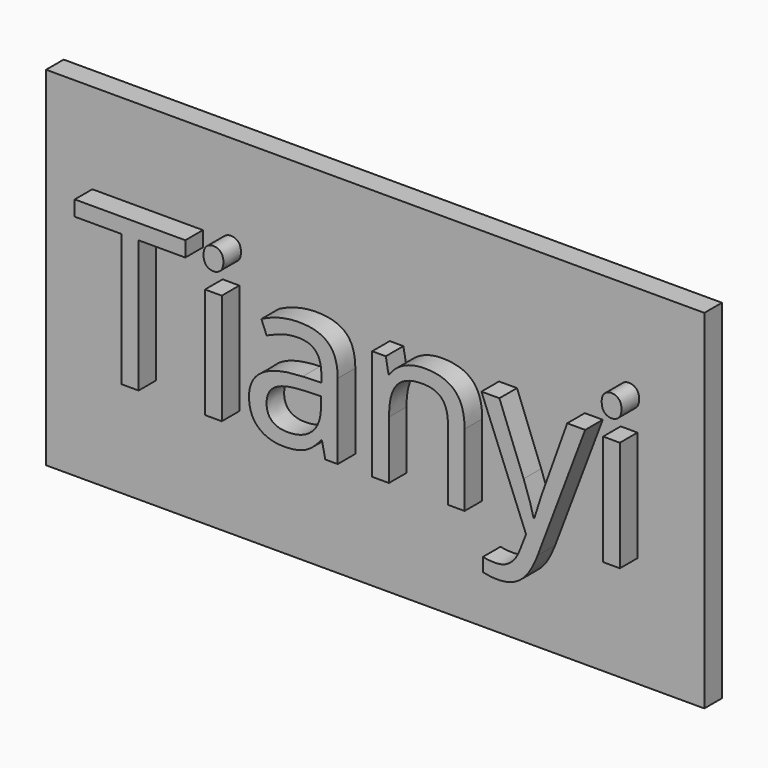
from build123d import *

# Parameters (mm, degrees)
F0_W         = 76.0509371758
F0_H         = 40.2351804078
F2_DEPTH     = 2.54
F1_TEXT_SIZE = 23.8719266943
F3_DEPTH     = 5.08


# Not quite as in the source:
# - Text() gives the source's letters only with a copy of the font that has no kerning and outlines rounded to 1/6400 em; it was checked with that copy


with BuildPart() as f2:
    # F0 (on Front) → F2 (new body)
    with BuildSketch(Plane.XZ):
        with Locations((38.0254685879, -20.1175902039)):
            Rectangle(F0_W, F0_H)
    extrude(amount=F2_DEPTH)

    # F1 (on face) → F3 (join)
    with BuildSketch(Plane.XZ):
        with Locations((5.1346663386, -27.4631232023)):
            Text('Tianyi', F1_TEXT_SIZE, font='Open Sans', text_align=(TextAlign.LEFT, TextAlign.BOTTOM))
    extrude(amount=F3_DEPTH)


solid = f2.part
